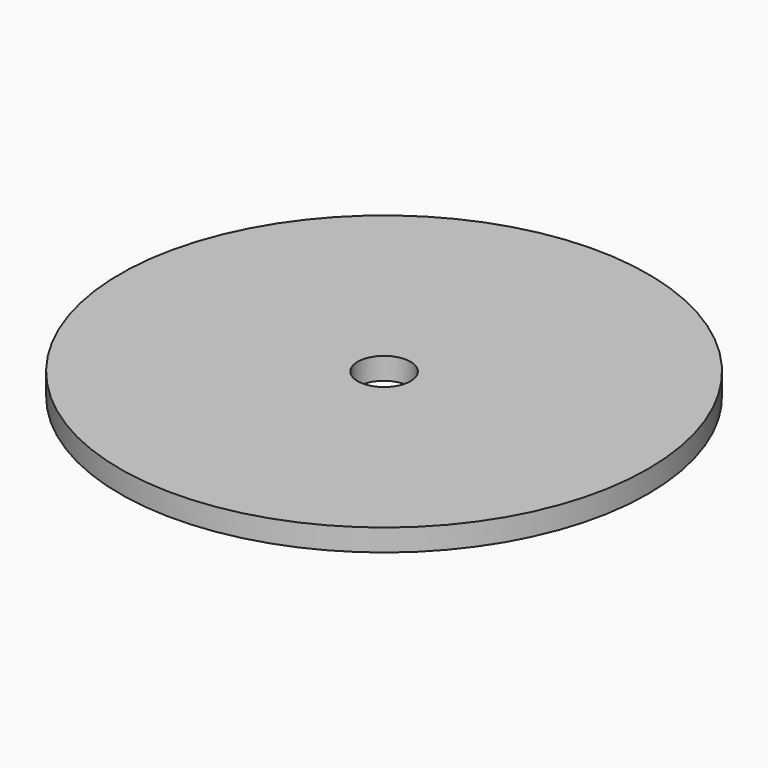
from build123d import *

# Parameters (mm, degrees)
F0_R     = 38.1
F0_R_2   = 3.81
F1_DEPTH = 3.175


# Not quite as in the source:
# - the program builds the solid bodies; features that only make, move or delete a surface that nothing else refers to are left out


with BuildPart() as f1:
    # F0 (on Top) → F1 (new body)
    with BuildSketch(Plane.XY):
        Circle(F0_R)
        Circle(F0_R_2, mode=Mode.SUBTRACT)
    extrude(amount=F1_DEPTH)


solid = f1.part
